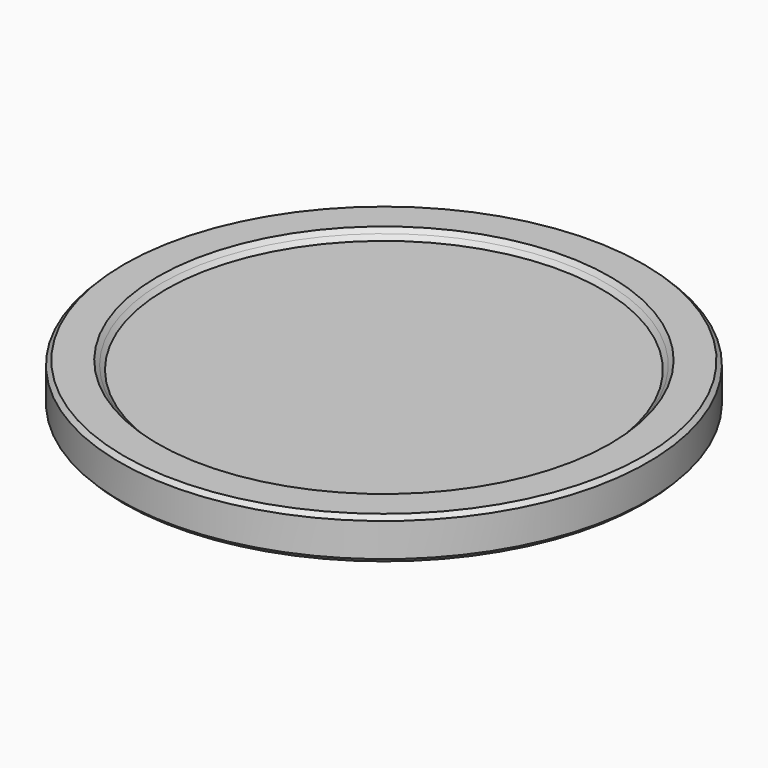
from build123d import *

# Parameters (mm, degrees)
F2_SIZE = 0.49999


# Not quite as in the source:
# - a fillet or chamfer is up to 0.001 mm smaller than in the source, because OpenCascade refuses the exact size


with BuildPart() as f1:
    # F0 (on Front) → F1 (revolve)
    with BuildSketch(Plane.XZ):
        Polygon((-31.5, 0), (0, 0), (0, 4), (-26.5, 4), (-26.5, 5), (-31.5, 5), align=None)
    revolve(axis=Axis((0, 0, 2), (0, 0, -1)))

    # F2 (size 0.5 in the source; OpenCascade refuses exactly that, so slightly less here)
    f2_edges = [f1.edges().sort_by_distance(p)[0] for p in [
        (26.5, 0, 4),
        (26.5, 0, 5),
        (31.5, 0, 5),
        (31.5, 0, 0),
    ]]
    chamfer(f2_edges, length=F2_SIZE)


solid = f1.part
